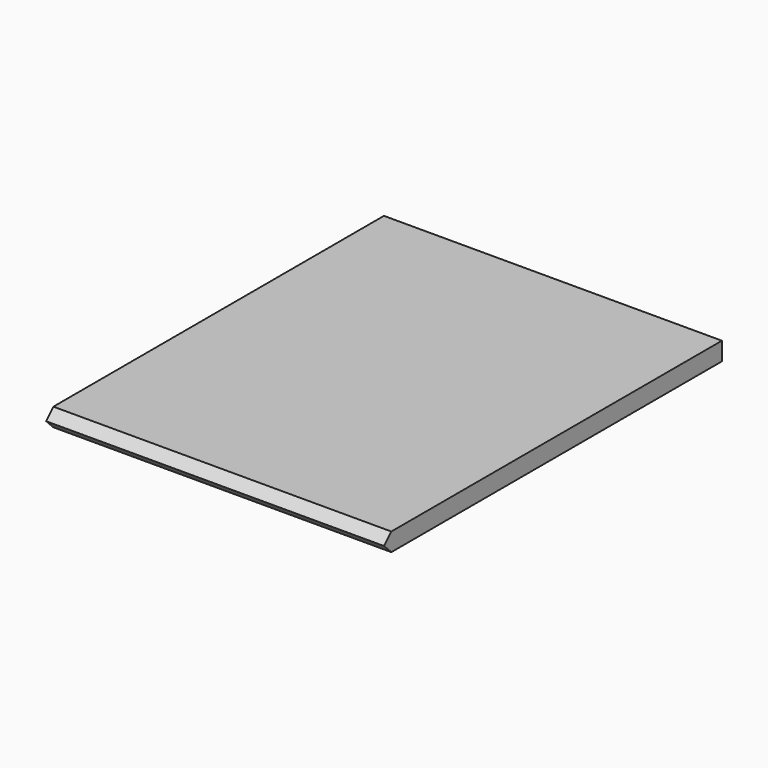
from build123d import *

# Parameters (mm, degrees)
F1_W          = 92.9454192519
F1_H          = 116.1409467459
F2_DEPTH      = 2.5
F2_DEPTH_BACK = 2.5
F3_SIZE       = 2.49999
F0_W          = 71.3404193521
F0_H          = 85.4026153684
F4_DEPTH      = 1
F4_DEPTH_BACK = 1


# Not quite as in the source:
# - a fillet or chamfer is up to 0.001 mm smaller than in the source, because OpenCascade refuses the exact size


with BuildPart() as f2:
    # F1 (on face) → F2 (new body, two sides)
    with BuildSketch(Plane.XY) as f2_sk:
        Rectangle(F1_W, F1_H)
    extrude(amount=F2_DEPTH)
    extrude(f2_sk.sketch, amount=-F2_DEPTH_BACK)

    # F3 (size 2.5 in the source; OpenCascade refuses exactly that, so slightly less here)
    f3_edges = [f2.edges().sort_by_distance(p)[0] for p in [
        (0, -58.070473, 2.5),
        (0, -58.070473, -2.5),
    ]]
    chamfer(f3_edges, length=F3_SIZE)

    # F0 (on Top) → F4 (join, two sides)
    with BuildSketch(Plane.XY) as f4_sk:
        Rectangle(F0_W, F0_H)
    extrude(amount=F4_DEPTH)
    extrude(f4_sk.sketch, amount=-F4_DEPTH_BACK)


solid = f2.part
